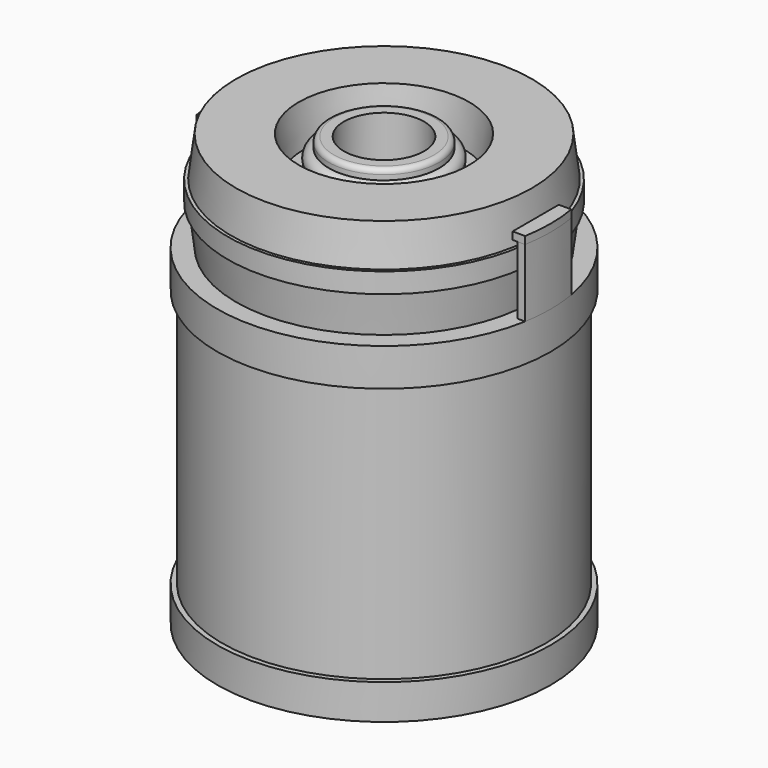
from build123d import *
from build123d import SkipClean  # not in build123d's __all__

# Parameters (mm, degrees)
F0_W     = 15
F0_H     = 51.5
F2_R     = 1.75
F5_DEPTH = 13.5
F7_DEPTH = 1.5


# Not quite as in the source:
# - after a boolean that leaves OpenCascade's solid faulty, fix() repairs it


with BuildPart() as f1:
    # F0 (on Front) → F1 (revolve)
    with BuildSketch(Plane.XZ):
        with BuildLine():
            Line((8, 17), (8, 0))
            Line((8, 0), (10, 0))
            ThreePointArc((10, 0), (10.7071067812, 0.2928932188), (11, 1))
            Line((11, 1), (11, 1.5))
            Line((11, 1.5), (9.25, 1.5))
            Line((9.25, 1.5), (9.25, 5))
            Line((9.25, 5), (11, 5))
            Line((11, 5), (11, 6.5))
            Line((11, 6.5), (9.25, 6.5))
            Line((9.25, 6.5), (9.25, 10))
            Line((9.25, 10), (33.25, 10))
            Line((33.25, 10), (33.25, 17))
            Line((33.25, 17), (32.25, 17))
            Line((32.25, 17), (17.25, 17))
            Line((17.25, 17), (8, 17))
        make_face()
        with Locations((24.75, 42.75)):
            Rectangle(F0_W, F0_H)
        with BuildLine():
            Line((8, 68.5), (17.25, 68.5))
            Line((17.25, 68.5), (32.25, 68.5))
            Line((32.25, 68.5), (33.25, 68.5))
            Line((33.25, 68.5), (33.25, 76))
            Line((33.25, 76), (16.5, 76))
            Line((16.5, 76), (9.25, 76))
            Line((9.25, 76), (9.25, 80.5))
            Line((9.25, 80.5), (16.5, 80.5))
            Line((16.5, 80.5), (16.5, 82.5))
            Line((16.5, 82.5), (13.127643615, 82.5))
            Line((13.127643615, 82.5), (9.25, 82.5))
            Line((9.25, 82.5), (9.25, 88))
            Line((9.25, 88), (11, 88))
            Line((11, 88), (11, 90))
            Line((11, 90), (9.25, 90))
            Line((9.25, 90), (9.25, 93.5))
            Line((9.25, 93.5), (11, 93.5))
            Line((11, 93.5), (11, 94.5))
            ThreePointArc((11, 94.5), (10.7071067812, 95.2071067812), (10, 95.5))
            Line((10, 95.5), (8, 95.5))
            Line((8, 95.5), (8, 68.5))
        make_face()
    revolve(axis=Axis((0, 0, 8.8243792458), (0, 0, 1)))

    # F4 (on face) → F5 (join)
    with BuildSketch(Plane.XY.offset(76)):
        with BuildLine():
            Line((31.224989992, -5.75), (32.7490457876, -5.75))
            ThreePointArc((32.7490457876, -5.75), (33.25, 0), (32.7490457876, 5.75))
            Line((32.7490457876, 5.75), (31.224989992, 5.75))
            ThreePointArc((31.224989992, 5.75), (31.75, 0), (31.224989992, -5.75))
        make_face()
        with BuildLine():
            Line((-31.224989992, 5.75), (-32.7490457876, 5.75))
            ThreePointArc((-32.7490457876, 5.75), (-33.25, 0), (-32.7490457876, -5.75))
            Line((-32.7490457876, -5.75), (-31.224989992, -5.75))
            ThreePointArc((-31.224989992, -5.75), (-31.75, 0), (-31.224989992, 5.75))
        make_face()
    with SkipClean():  # cleaning this boolean's faces spoils the solid; the shape is the same uncleaned
        extrude(amount=F5_DEPTH)

    # F6 (on face) → F7 (join)
    with BuildSketch(Plane.XY.offset(89.5)):
        with BuildLine():
            ThreePointArc((32.7490457876, -5.75), (33.25, 0), (32.7490457876, 5.75))
            Line((32.7490457876, 5.75), (30.25, 5.75))
            Line((30.25, 5.75), (30.25, -5.75))
            Line((30.25, -5.75), (32.7490457876, -5.75))
        make_face()
        with BuildLine():
            ThreePointArc((-32.7490457876, 5.75), (-33.25, 0), (-32.7490457876, -5.75))
            Line((-32.7490457876, -5.75), (-30.25, -5.75))
            Line((-30.25, -5.75), (-30.25, 5.75))
            Line((-30.25, 5.75), (-32.7490457876, 5.75))
        make_face()
    extrude(amount=F7_DEPTH)

    add(f1.part.fix(), mode=Mode.REPLACE)


with BuildPart() as f3:
    # F2 (on Front) → F3 (revolve)
    with BuildSketch(Plane.XZ):
        with Locations((11, 91.75)):
            Circle(F2_R)
    revolve(axis=Axis((0, 0, 8.8243792458), (0, 0, 1)))


with BuildPart() as f3b:
    # F2 (on Front) → F3, piece 2 (revolve)
    with BuildSketch(Plane.XZ):
        with Locations((11, 3.25)):
            Circle(F2_R)
    revolve(axis=Axis((0, 0, 8.8243792458), (0, 0, 1)))


with BuildPart() as f9:
    # F8 (on Front) → F9 (revolve)
    with BuildSketch(Plane.XZ):
        Polygon((-30.5, 84), (-29.5, 76), (-17, 76), (-16, 84), (-13.5, 84), (-13.5, 86), (-31.1389584094, 86), (-31.1389584094, 84), align=None)
        Polygon((-31.1389584094, 88), (-31.1389584094, 86), (-13.5, 86), (-13.5, 88), (-16, 88), (-17, 96), (-29.5, 96), (-30.5, 88), align=None)
    revolve(axis=Axis((0, 0, 47.1165850759), (0, 0, 1)))


solid = Compound([f1.part, f3.part, f3b.part, f9.part])
